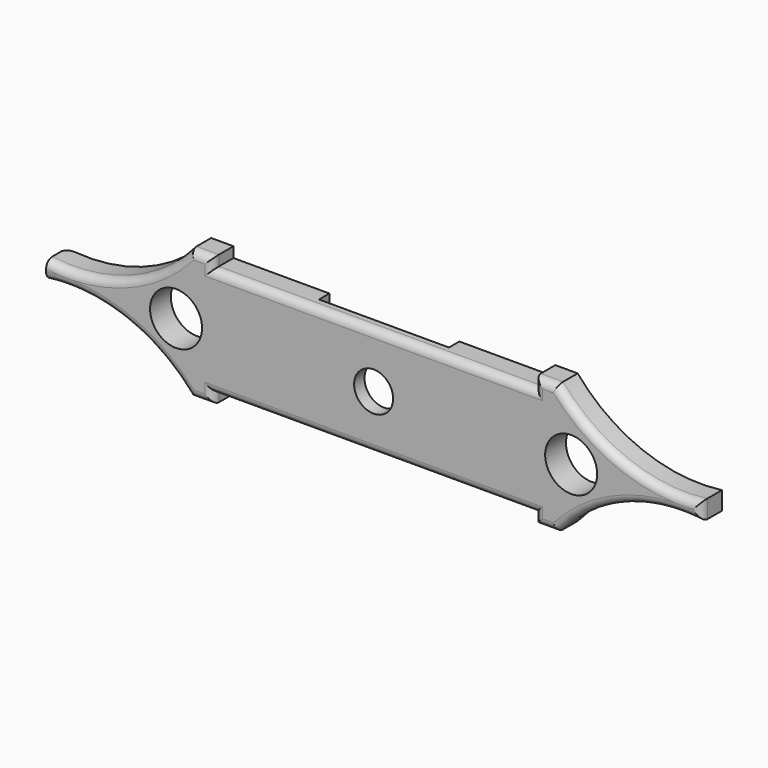
from build123d import *

# Parameters (mm, degrees)
F0_R         = 10
F0_R_2       = 7.5
F1_DEPTH     = 10
F2_W         = 50
F2_H         = 42
F2_R         = 7.5
F3_DEPTH     = 5
F4_T1_DEPTH  = 123.8
F4_T3_DEPTH  = 11.5
F4_T5_DEPTH  = 23.6
F4_T7_DEPTH  = 22
F4_T9_DEPTH  = 11.5
F4_T11_DEPTH = 23.6
F4_T14_ANGLE = 71.0490813257
F4_T16_ANGLE = 71.0490813257
F4_T18_ANGLE = 71.0490813257
F4_T20_ANGLE = 71.0490813257
F4_T25_DEPTH = 19
F4_T29_DEPTH = 131.3
F4_T36_DEPTH = 131.3
F4_T40_DEPTH = 19
F4_T47_DEPTH = 19
F4_T51_DEPTH = 131.3
F4_T58_DEPTH = 131.3
F4_T62_DEPTH = 19


# Not quite as in the source:
# - a fillet or chamfer that OpenCascade refuses, or shapes differently, is made with other operations: its cross-section is extruded or revolved along the edge and cut away or added


with BuildPart() as f1:
    # F0 (on Front) → F1 (new body)
    with BuildSketch(Plane.XZ):
        with BuildLine():
            ThreePointArc((126, 3.5), (95.5089399385, 7.1742403064), (70.5, 25))
            Line((70.5, 25), (61.9, 25))
            Line((61.9, 25), (61.9, 21))
            Line((61.9, 21), (-61.9, 21))
            Line((-61.9, 21), (-61.9, 25))
            Line((-61.9, 25), (-70.5, 25))
            ThreePointArc((-70.5, 25), (-95.5089399385, 7.1742403064), (-126, 3.5))
            Line((-126, 3.5), (-126, -3.5))
            ThreePointArc((-126, -3.5), (-95.5089399385, -7.1742403064), (-70.5, -25))
            Line((-70.5, -25), (-61.9, -25))
            Line((-61.9, -25), (-61.9, -21))
            Line((-61.9, -21), (61.9, -21))
            Line((61.9, -21), (61.9, -25))
            Line((61.9, -25), (70.5, -25))
            ThreePointArc((70.5, -25), (95.5089399385, -7.1742403064), (126, -3.5))
            Line((126, -3.5), (126, 3.5))
        make_face()
        with Locations((-76, 0)):
            Circle(F0_R, mode=Mode.SUBTRACT)
        Circle(F0_R_2, mode=Mode.SUBTRACT)
        with Locations((76, 0)):
            Circle(F0_R, mode=Mode.SUBTRACT)
    extrude(amount=F1_DEPTH)

    # F2 (on face) → F3 (cut)
    with BuildSketch(Plane(origin=(0, 0, 0), x_dir=(-1, 0, 0), z_dir=(0, 1, 0))):
        Rectangle(F2_W, F2_H)
        Circle(F2_R, mode=Mode.SUBTRACT)
    extrude(amount=-F3_DEPTH, mode=Mode.SUBTRACT)

    # F4: fillet of radius 3 on 16 edges, made by hand

    # F4_s2 → F4_t1 (cut)
    with BuildSketch(Plane.YZ.offset(-61.9)):
        with BuildLine():
            ThreePointArc((-10, -18), (-9.1213203436, -20.1213203436), (-7, -21))
            Line((-7, -21), (-10, -21))
            Line((-10, -21), (-10, -18))
        make_face()
        with BuildLine():
            ThreePointArc((-10, 18), (-9.1213203436, 20.1213203436), (-7, 21))
            Line((-7, 21), (-10, 21))
            Line((-10, 21), (-10, 18))
        make_face()
    extrude(amount=F4_T1_DEPTH, mode=Mode.SUBTRACT)

    # F4_s4 → F4_t3 (cut)
    with BuildSketch(Plane.XY.offset(-32.5)):
        with BuildLine():
            ThreePointArc((64.9, -10), (62.7786796564, -9.1213203436), (61.9, -7))
            Line((61.9, -7), (61.9, -10))
            Line((61.9, -10), (64.9, -10))
        make_face()
        with BuildLine():
            ThreePointArc((-64.9, -10), (-62.7786796564, -9.1213203436), (-61.9, -7))
            Line((-61.9, -7), (-61.9, -10))
            Line((-61.9, -10), (-64.9, -10))
        make_face()
    extrude(amount=F4_T3_DEPTH, mode=Mode.SUBTRACT)

    # F4_s6 → F4_t5 (cut)
    with BuildSketch(Plane.YZ.offset(54.4)):
        with BuildLine():
            ThreePointArc((-10, -22), (-9.1213203436, -24.1213203436), (-7, -25))
            Line((-7, -25), (-10, -25))
            Line((-10, -25), (-10, -22))
        make_face()
        with BuildLine():
            ThreePointArc((-10, 22), (-9.1213203436, 24.1213203436), (-7, 25))
            Line((-7, 25), (-10, 25))
            Line((-10, 25), (-10, 22))
        make_face()
    extrude(amount=F4_T5_DEPTH, mode=Mode.SUBTRACT)

    # F4_s8 → F4_t7 (cut)
    with BuildSketch(Plane.XY.offset(-11)):
        with BuildLine():
            ThreePointArc((123, -10), (125.1213203436, -9.1213203436), (126, -7))
            Line((126, -7), (126, -10))
            Line((126, -10), (123, -10))
        make_face()
        with BuildLine():
            ThreePointArc((-123, 0), (-125.1213203436, -0.8786796564), (-126, -3))
            Line((-126, -3), (-126, 0))
            Line((-126, 0), (-123, 0))
        make_face()
    extrude(amount=F4_T7_DEPTH, mode=Mode.SUBTRACT)

    # F4_s10 → F4_t9 (cut)
    with BuildSketch(Plane.XY.offset(21)):
        with BuildLine():
            ThreePointArc((64.9, -10), (62.7786796564, -9.1213203436), (61.9, -7))
            Line((61.9, -7), (61.9, -10))
            Line((61.9, -10), (64.9, -10))
        make_face()
        with BuildLine():
            ThreePointArc((-64.9, -10), (-62.7786796564, -9.1213203436), (-61.9, -7))
            Line((-61.9, -7), (-61.9, -10))
            Line((-61.9, -10), (-64.9, -10))
        make_face()
    extrude(amount=F4_T9_DEPTH, mode=Mode.SUBTRACT)

    # F4_s12 → F4_t11 (cut)
    with BuildSketch(Plane.YZ.offset(-78)):
        with BuildLine():
            ThreePointArc((-10, 22), (-9.1213203436, 24.1213203436), (-7, 25))
            Line((-7, 25), (-10, 25))
            Line((-10, 25), (-10, 22))
        make_face()
        with BuildLine():
            ThreePointArc((-10, -22), (-9.1213203436, -24.1213203436), (-7, -25))
            Line((-7, -25), (-10, -25))
            Line((-10, -25), (-10, -22))
        make_face()
    extrude(amount=F4_T11_DEPTH, mode=Mode.SUBTRACT)

    # F4_s13 → F4_t14 (revolve, cut)
    with BuildSketch(Plane(origin=(5.6700188901, 0, 8.6318707647), x_dir=(0, 1, 0), z_dir=(-0.5490187323, 0, -0.8358100452))):
        with BuildLine():
            ThreePointArc((-10, 69.1979444633), (-9.1213203436, 71.3192648069), (-7, 72.1979444633))
            Line((-7, 72.1979444633), (-10, 72.1979444633))
            Line((-10, 72.1979444633), (-10, 69.1979444633))
        make_face()
    revolve(axis=Axis((117.9593619468, -10, -65.127655258), (0, 1, 0)), revolution_arc=F4_T14_ANGLE, mode=Mode.SUBTRACT)

    # F4_s15 → F4_t16 (revolve, cut)
    with BuildSketch(Plane(origin=(126.3513869763, 0, 32.3212006938), x_dir=(0, 1, 0), z_dir=(0.9688050004, 0, 0.2478242748))):
        with BuildLine():
            ThreePointArc((-7, -28.2871731549), (-9.1213203436, -29.1658528113), (-10, -31.2871731549))
            Line((-10, -31.2871731549), (-10, -28.2871731549))
            Line((-10, -28.2871731549), (-7, -28.2871731549))
        make_face()
    revolve(axis=Axis((117.9593619468, -10, 65.127655258), (0, 1, 0)), revolution_arc=F4_T16_ANGLE, mode=Mode.SUBTRACT)

    # F4_s17 → F4_t18 (revolve, cut)
    with BuildSketch(Plane(origin=(-5.6700188901, 0, -8.6318707647), x_dir=(0, 1, 0), z_dir=(0.5490187323, 0, 0.8358100452))):
        with BuildLine():
            ThreePointArc((-10, 69.1979444633), (-9.1213203436, 71.3192648069), (-7, 72.1979444633))
            Line((-7, 72.1979444633), (-10, 72.1979444633))
            Line((-10, 72.1979444633), (-10, 69.1979444633))
        make_face()
    revolve(axis=Axis((-117.9593619468, -10, 65.127655258), (0, 1, 0)), revolution_arc=F4_T18_ANGLE, mode=Mode.SUBTRACT)

    # F4_s19 → F4_t20 (revolve, cut)
    with BuildSketch(Plane(origin=(-126.3513869763, 0, -32.3212006938), x_dir=(0, 1, 0), z_dir=(-0.9688050004, 0, -0.2478242748))):
        with BuildLine():
            ThreePointArc((-10, -31.2871731549), (-9.1213203436, -29.1658528113), (-7, -28.2871731549))
            Line((-7, -28.2871731549), (-10, -28.2871731549))
            Line((-10, -28.2871731549), (-10, -31.2871731549))
        make_face()
    revolve(axis=Axis((-117.9593619468, -10, -65.127655258), (0, 1, 0)), revolution_arc=F4_T20_ANGLE, mode=Mode.SUBTRACT)


with BuildPart() as f4_tool23:
    # F4_s24 → F4_t25 (new body)
    with BuildSketch(Plane.XY.offset(-32.5)):
        with BuildLine():
            ThreePointArc((-64.9, -10), (-62.7786796564, -9.1213203436), (-61.9, -7))
            Line((-61.9, -7), (-61.9, -10))
            Line((-61.9, -10), (-64.9, -10))
        make_face()
    extrude(amount=F4_T25_DEPTH)

    split(bisect_by=Plane.XY.offset(-21), keep=Keep.TOP)


with BuildPart() as f4_tool27:
    # F4_s28 → F4_t29 (new body)
    with BuildSketch(Plane.YZ.offset(-69.4)):
        with BuildLine():
            ThreePointArc((-10, -18), (-9.1213203436, -20.1213203436), (-7, -21))
            Line((-7, -21), (-10, -21))
            Line((-10, -21), (-10, -18))
        make_face()
    extrude(amount=F4_T29_DEPTH)

    split(bisect_by=Plane.YZ.offset(-61.9), keep=Keep.BOTTOM)


with BuildPart() as f4_tool23_1:
    add(f4_tool23.part)

    # F4_t31: intersect F4_tool27
    add(f4_tool27.part, mode=Mode.INTERSECT)


with BuildPart() as f1_1:
    add(f1.part)

    # F4_t21: cut F4_tool23
    add(f4_tool23_1.part, mode=Mode.SUBTRACT)


with BuildPart() as f4_tool34:
    # F4_s35 → F4_t36 (new body)
    with BuildSketch(Plane.YZ.offset(-61.9)):
        with BuildLine():
            ThreePointArc((-10, -18), (-9.1213203436, -20.1213203436), (-7, -21))
            Line((-7, -21), (-10, -21))
            Line((-10, -21), (-10, -18))
        make_face()
    extrude(amount=F4_T36_DEPTH)

    split(bisect_by=Plane.YZ.offset(61.9), keep=Keep.TOP)


with BuildPart() as f4_tool38:
    # F4_s39 → F4_t40 (new body)
    with BuildSketch(Plane.XY.offset(-13.5)):
        with BuildLine():
            ThreePointArc((64.9, -10), (62.7786796564, -9.1213203436), (61.9, -7))
            Line((61.9, -7), (61.9, -10))
            Line((61.9, -10), (64.9, -10))
        make_face()
    extrude(amount=-F4_T40_DEPTH)

    split(bisect_by=Plane.XY.offset(-21), keep=Keep.TOP)


with BuildPart() as f4_tool34_1:
    add(f4_tool34.part)

    # F4_t42: intersect F4_tool38
    add(f4_tool38.part, mode=Mode.INTERSECT)


with BuildPart() as f1_2:
    add(f1_1.part)

    # F4_t32: cut F4_tool34
    add(f4_tool34_1.part, mode=Mode.SUBTRACT)


with BuildPart() as f4_tool45:
    # F4_s46 → F4_t47 (new body)
    with BuildSketch(Plane.XY.offset(32.5)):
        with BuildLine():
            ThreePointArc((64.9, -10), (62.7786796564, -9.1213203436), (61.9, -7))
            Line((61.9, -7), (61.9, -10))
            Line((61.9, -10), (64.9, -10))
        make_face()
    extrude(amount=-F4_T47_DEPTH)

    split(bisect_by=Plane.XY.offset(21), keep=Keep.BOTTOM)


with BuildPart() as f4_tool49:
    # F4_s50 → F4_t51 (new body)
    with BuildSketch(Plane.YZ.offset(69.4)):
        with BuildLine():
            ThreePointArc((-10, 18), (-9.1213203436, 20.1213203436), (-7, 21))
            Line((-7, 21), (-10, 21))
            Line((-10, 21), (-10, 18))
        make_face()
    extrude(amount=-F4_T51_DEPTH)

    split(bisect_by=Plane.YZ.offset(61.9), keep=Keep.TOP)


with BuildPart() as f4_tool45_1:
    add(f4_tool45.part)

    # F4_t53: intersect F4_tool49
    add(f4_tool49.part, mode=Mode.INTERSECT)


with BuildPart() as f1_3:
    add(f1_2.part)

    # F4_t43: cut F4_tool45
    add(f4_tool45_1.part, mode=Mode.SUBTRACT)


with BuildPart() as f4_tool56:
    # F4_s57 → F4_t58 (new body)
    with BuildSketch(Plane.YZ.offset(61.9)):
        with BuildLine():
            ThreePointArc((-10, 18), (-9.1213203436, 20.1213203436), (-7, 21))
            Line((-7, 21), (-10, 21))
            Line((-10, 21), (-10, 18))
        make_face()
    extrude(amount=-F4_T58_DEPTH)

    split(bisect_by=Plane.YZ.offset(-61.9), keep=Keep.BOTTOM)


with BuildPart() as f4_tool60:
    # F4_s61 → F4_t62 (new body)
    with BuildSketch(Plane.XY.offset(13.5)):
        with BuildLine():
            ThreePointArc((-64.9, -10), (-62.7786796564, -9.1213203436), (-61.9, -7))
            Line((-61.9, -7), (-61.9, -10))
            Line((-61.9, -10), (-64.9, -10))
        make_face()
    extrude(amount=F4_T62_DEPTH)

    split(bisect_by=Plane.XY.offset(21), keep=Keep.BOTTOM)


with BuildPart() as f4_tool56_1:
    add(f4_tool56.part)

    # F4_t64: intersect F4_tool60
    add(f4_tool60.part, mode=Mode.INTERSECT)


with BuildPart() as f1_4:
    add(f1_3.part)

    # F4_t54: cut F4_tool56
    add(f4_tool56_1.part, mode=Mode.SUBTRACT)


solid = f1_4.part
